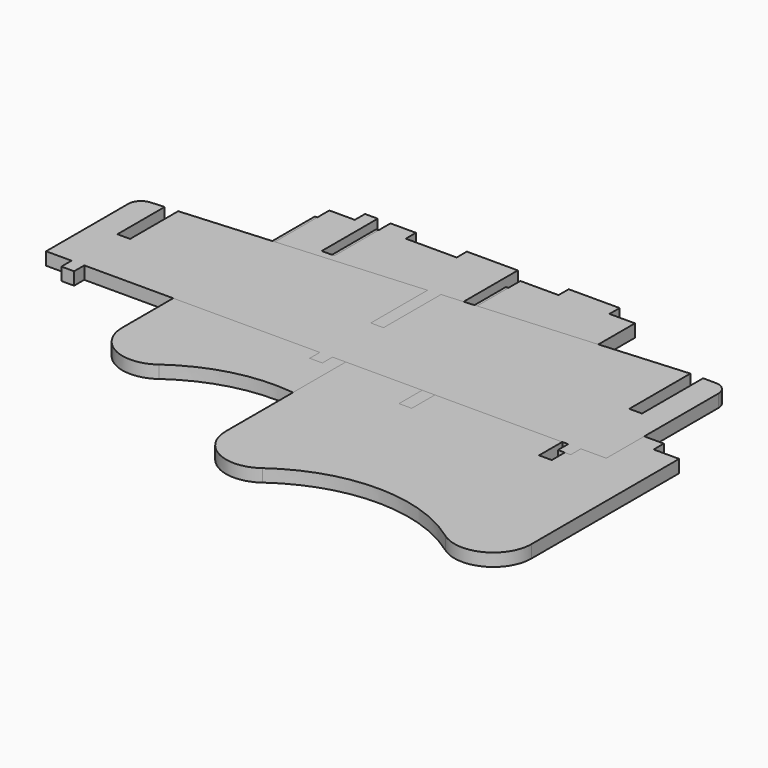
from build123d import *

# Parameters (mm, degrees)
F5_DEPTH = 5
F6_DEPTH = 5
F7_DEPTH = 5
F8_DEPTH = 5


# Not quite as in the source:
# - the dataset's text gives a spline's control points without its knots; the knots are read off the source's solid


with BuildPart() as f5:
    # F1 (on Top) → F5 (new body)
    with BuildSketch(Plane.XY):
        with BuildLine():
            add(Edge.make_bspline(
                [(35.7727633026, -67.1033849488), (33.1888546546, -65.2263313398), (27.7258131524, -61.8786878763), (18.8464933001, -58.2010364024), (9.5012368587, -55.9575441024), (-0.0799322126, -55.2035239896), (-9.661101284, -55.9575441023), (-19.0063577254, -58.2010364023), (-27.8856775777, -61.8786878761), (-33.3487190799, -65.2263313396), (-35.932627728, -67.1033849485)],
                knots=[0.2739165322, 0.2739165322, 0.2739165322, 0.2739165322, 0.3304373991, 0.3869582661, 0.443479133, 0.5, 0.556520867, 0.6130417339, 0.6695626009, 0.7260834678, 0.7260834678, 0.7260834678, 0.7260834678], degree=3))
            add(Edge.make_bspline(
                [(35.7727633017, -67.1033849481), (59.9200677872, -84.6449435725), (59.9200677872, -55.0144236535)],
                knots=[0.9372459818, 0.9372459818, 0.9372459818, 3.1415926536, 3.1415926536, 3.1415926536], degree=2, weights=[1, 0.4516581587, 1]))
            Line((59.9200677872, -55.0144236535), (59.9200677872, 39.5451359728))
            Line((59.9200677872, 39.5451359728), (49.9200677872, 39.5451359728))
            Line((49.9200677872, 39.5451359728), (49.9200677872, 44.5451359728))
            Line((49.9200677872, 44.5451359728), (29.9200677872, 44.5451359728))
            Line((29.9200677872, 44.5451359728), (29.9200677872, 39.5451359728))
            Line((29.9200677872, 39.5451359728), (14.9200677872, 39.5451359728))
            Line((14.9200677872, 39.5451359728), (14.9200677872, 9.5451359728))
            Line((14.9200677872, 9.5451359728), (9.9200677872, 9.5451359728))
            Line((9.9200677872, 9.5451359728), (9.9200677872, 39.5451359728))
            Line((9.9200677872, 39.5451359728), (9.9200677872, 44.5451359728))
            Line((9.9200677872, 44.5451359728), (-10.0799322128, 44.5451359728))
            Line((-10.0799322128, 44.5451359728), (-10.0799322128, 39.5451359728))
            Line((-10.0799322128, 39.5451359728), (-30.0799322128, 39.5451359728))
            Line((-30.0799322128, 39.5451359728), (-30.0799322128, 44.5451359728))
            Line((-30.0799322128, 44.5451359728), (-40.0799322128, 44.5451359728))
            Line((-40.0799322128, 44.5451359728), (-40.0799322128, 9.5451359728))
            Line((-40.0799322128, 9.5451359728), (-45.0799322128, 9.5451359728))
            Line((-45.0799322128, 9.5451359728), (-45.0799322128, 39.5451359728))
            Line((-45.0799322128, 39.5451359728), (-45.0799322128, 44.5451359728))
            Line((-45.0799322128, 44.5451359728), (-50.0799322128, 44.5451359728))
            Line((-50.0799322128, 44.5451359728), (-50.0799322128, 39.5451359728))
            Line((-50.0799322128, 39.5451359728), (-60.0799322128, 39.5451359728))
            Line((-60.0799322128, 39.5451359728), (-60.0799322128, -55.0144236535))
            add(Edge.make_bspline(
                [(-60.0799322128, -55.0144236535), (-60.0799322128, -84.6449435725), (-35.9326277274, -67.1033849481)],
                knots=[0, 0, 0, 2.2043466718, 2.2043466718, 2.2043466718], degree=2, weights=[1, 0.4516581587, 1]))
        make_face()
    extrude(amount=F5_DEPTH)


with BuildPart() as f6:
    # F2 (on Top) → F6 (new body)
    with BuildSketch(Plane.XY):
        with BuildLine():
            add(Edge.make_bspline(
                [(103.5514379038, -100.9854254094), (100.9675292558, -99.1083718005), (95.5044877536, -95.760728337), (86.6251679013, -92.083076863), (77.2799114599, -89.8395845631), (67.6987423886, -89.0855644503), (58.1175733172, -89.839584563), (48.7723168758, -92.0830768629), (39.8929970235, -95.7607283368), (34.4299555213, -99.1083718002), (31.8460468732, -100.9854254092)],
                knots=[0.2739165322, 0.2739165322, 0.2739165322, 0.2739165322, 0.3304373991, 0.3869582661, 0.443479133, 0.5, 0.556520867, 0.6130417339, 0.6695626009, 0.7260834678, 0.7260834678, 0.7260834678, 0.7260834678], degree=3))
            add(Edge.make_bspline(
                [(103.5514379029, -100.9854254088), (127.6987423883, -118.5269840331), (127.6987423883, -88.8964641141)],
                knots=[0.9372459818, 0.9372459818, 0.9372459818, 3.1415926536, 3.1415926536, 3.1415926536], degree=2, weights=[1, 0.4516581587, 1]))
            Line((127.6987423883, -88.8964641141), (127.6987423883, -16.3964641141))
            Line((127.6987423883, -16.3964641141), (117.6987423883, -16.3964641141))
            Line((117.6987423883, -16.3964641141), (117.6987423883, -11.3964641141))
            Line((117.6987423883, -11.3964641141), (97.6987423883, -11.3964641141))
            Line((97.6987423883, -11.3964641141), (97.6987423883, -41.3964641141))
            Line((97.6987423883, -41.3964641141), (92.6987423883, -41.3964641141))
            Line((92.6987423883, -41.3964641141), (92.6987423883, -16.3964641141))
            Line((92.6987423883, -16.3964641141), (77.6987423883, -16.3964641141))
            Line((77.6987423883, -16.3964641141), (77.6987423883, -11.3964641141))
            Line((77.6987423883, -11.3964641141), (57.6987423883, -11.3964641141))
            Line((57.6987423883, -11.3964641141), (57.6987423883, -16.3964641141))
            Line((57.6987423883, -16.3964641141), (42.6987423883, -16.3964641141))
            Line((42.6987423883, -16.3964641141), (42.6987423883, -41.3964641141))
            Line((42.6987423883, -41.3964641141), (37.6987423883, -41.3964641141))
            Line((37.6987423883, -41.3964641141), (37.6987423883, -11.3964641141))
            Line((37.6987423883, -11.3964641141), (17.6987423883, -11.3964641141))
            Line((17.6987423883, -11.3964641141), (17.6987423883, -16.3964641141))
            Line((17.6987423883, -16.3964641141), (7.6987423883, -16.3964641141))
            Line((7.6987423883, -16.3964641141), (7.6987423883, -88.8964641141))
            add(Edge.make_bspline(
                [(7.6987423883, -88.8964641141), (7.6987423883, -118.5269840331), (31.8460468738, -100.9854254088)],
                knots=[0, 0, 0, 2.2043466718, 2.2043466718, 2.2043466718], degree=2, weights=[1, 0.4516581587, 1]))
        make_face()
    extrude(amount=F6_DEPTH)


with BuildPart() as f7:
    # F4 (on Top) → F7 (new body)
    with BuildSketch(Plane.XY):
        with BuildLine():
            add(Edge.make_bspline(
                [(36.7376570142, -21.649473493), (34.1537483662, -19.772419884), (28.690706864, -16.4247764205), (19.8113870117, -12.7471249466), (10.4661305703, -10.5036326466), (0.884961499, -9.7496125338), (-8.6962075724, -10.5036326465), (-18.0414640138, -12.7471249464), (-26.9207838661, -16.4247764203), (-32.3838253683, -19.7724198838), (-34.9677340164, -21.6494734927)],
                knots=[0.2739165322, 0.2739165322, 0.2739165322, 0.2739165322, 0.3304373991, 0.3869582661, 0.443479133, 0.5, 0.556520867, 0.6130417339, 0.6695626009, 0.7260834678, 0.7260834678, 0.7260834678, 0.7260834678], degree=3))
            add(Edge.make_bspline(
                [(36.7376570133, -21.6494734923), (60.8849614988, -39.1910321167), (60.8849614988, -9.5605121977)],
                knots=[0.9372459818, 0.9372459818, 0.9372459818, 3.1415926536, 3.1415926536, 3.1415926536], degree=2, weights=[1, 0.4516581587, 1]))
            Line((60.8849614988, -9.5605121977), (60.8849614988, 45.4394878023))
            Line((60.8849614988, 45.4394878023), (50.8849614988, 45.4394878023))
            Line((50.8849614988, 45.4394878023), (50.8849614988, 50.4394878023))
            Line((50.8849614988, 50.4394878023), (30.8849614988, 50.4394878023))
            Line((30.8849614988, 50.4394878023), (30.8849614988, 45.4394878023))
            Line((30.8849614988, 45.4394878023), (15.8849614988, 45.4394878023))
            Line((15.8849614988, 45.4394878023), (15.8849614988, 22.9394878023))
            Line((15.8849614988, 22.9394878023), (10.8849614988, 22.9394878023))
            Line((10.8849614988, 22.9394878023), (10.8849614988, 45.4394878023))
            Line((10.8849614988, 45.4394878023), (10.8849614988, 50.4394878023))
            Line((10.8849614988, 50.4394878023), (-9.1150385012, 50.4394878023))
            Line((-9.1150385012, 50.4394878023), (-9.1150385012, 45.4394878023))
            Line((-9.1150385012, 45.4394878023), (-29.1150385012, 45.4394878023))
            Line((-29.1150385012, 45.4394878023), (-29.1150385012, 50.4394878023))
            Line((-29.1150385012, 50.4394878023), (-39.1150385012, 50.4394878023))
            Line((-39.1150385012, 50.4394878023), (-39.1150385012, 22.9394878023))
            Line((-39.1150385012, 22.9394878023), (-44.1150385012, 22.9394878023))
            Line((-44.1150385012, 22.9394878023), (-44.1150385012, 45.4394878023))
            Line((-44.1150385012, 45.4394878023), (-44.1150385012, 50.4394878023))
            Line((-44.1150385012, 50.4394878023), (-49.1150385012, 50.4394878023))
            Line((-49.1150385012, 50.4394878023), (-49.1150385012, 45.4394878023))
            Line((-49.1150385012, 45.4394878023), (-59.1150385012, 45.4394878023))
            Line((-59.1150385012, 45.4394878023), (-59.1150385012, -9.5605121977))
            add(Edge.make_bspline(
                [(-59.1150385012, -9.5605121977), (-59.1150385012, -39.1910321167), (-34.9677340158, -21.6494734923)],
                knots=[0, 0, 0, 2.2043466718, 2.2043466718, 2.2043466718], degree=2, weights=[1, 0.4516581587, 1]))
        make_face()
    extrude(amount=F7_DEPTH)


with BuildPart() as f8:
    # F3 (on Top) → F8 (new body)
    with BuildSketch(Plane.XY):
        with BuildLine():
            Line((100, -30), (110, -30))
            Line((110, -30), (110, 25))
            ThreePointArc((110, 25), (108.5355339059, 28.5355339059), (105, 30))
            Line((105, 30), (100, 30))
            Line((100, 30), (100, 0))
            Line((100, 0), (95, 0))
            Line((95, 0), (95, 30))
            Line((95, 30), (2.5, 23.2317073171))
            Line((2.5, 23.2317073171), (2.5, -5))
            Line((2.5, -5), (-2.5, -5))
            Line((-2.5, -5), (-2.5, 22.8658536585))
            Line((-2.5, 22.8658536585), (-95, 16.0975609756))
            Line((-95, 16.0975609756), (-95, -7.5))
            Line((-95, -7.5), (-100, -7.5))
            Line((-100, -7.5), (-100, 15.7317073171))
            Line((-100, 15.7317073171), (-105.3648781916, 15.3391552543))
            ThreePointArc((-105.3648781916, 15.3391552543), (-108.6622664402, 13.7565730807), (-110, 10.3524866363))
            Line((-110, 10.3524866363), (-110, -30))
            Line((-110, -30), (-100, -30))
            Line((-100, -30), (-100, -35))
            Line((-100, -35), (-95, -35))
            Line((-95, -35), (-95, -30))
            Line((-95, -30), (-2.5, -30))
            Line((-2.5, -30), (-2.5, -35))
            Line((-2.5, -35), (2.5, -35))
            Line((2.5, -35), (2.5, -30))
            Line((2.5, -30), (95, -30))
            Line((95, -30), (95, -35))
            Line((95, -35), (100, -35))
            Line((100, -35), (100, -30))
        make_face()
    extrude(amount=F8_DEPTH)


solid = Compound([f5.part, f6.part, f7.part, f8.part])
